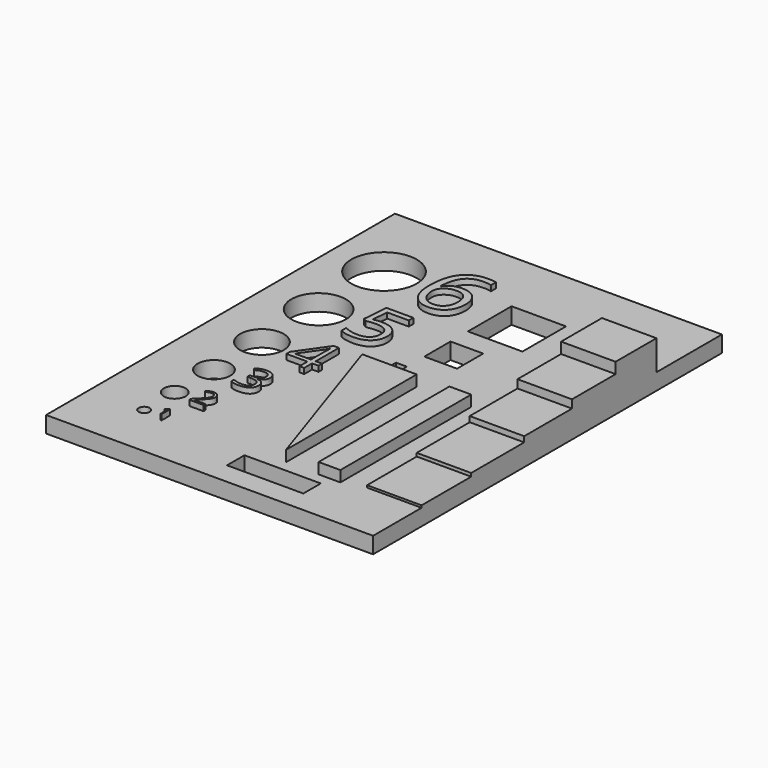
from build123d import *

# Parameters (mm, degrees)
F0_W           = 30
F0_H           = 40
F0_R           = 0.5
F0_R_2         = 1
F0_R_3         = 1.5
F0_R_4         = 2
F0_W_2         = 7
F0_H_2         = 2
F0_R_5         = 2.5
F0_R_6         = 3
F0_W_3         = 1
F0_H_3         = 1
F0_W_4         = 3
F0_H_4         = 3
F0_W_5         = 5
F0_H_5         = 5
F1_DEPTH       = 1.5
F3_DEPTH       = 5
F4_TEXT_SIZE   = 8.3333333333
F4_TEXT_SIZE_2 = 6.9444444444
F4_TEXT_SIZE_3 = 5.5555555556
F4_TEXT_SIZE_4 = 4.1666666667
F4_TEXT_SIZE_5 = 2.7777777778
F4_TEXT_SIZE_6 = 1.3888888889
F5_DEPTH       = 0.5
F6_W           = 2
F6_H           = 15
F7_DEPTH       = 1


# Not quite as in the source:
# - Text() gives the source's letters only with a copy of the font that has no kerning and outlines rounded to 1/6400 em; it was checked with that copy


with BuildPart() as f1:
    # F0 (on Top) → F1 (new body)
    with BuildSketch(Plane.XY):
        Rectangle(F0_W, F0_H)
        with Locations((-10, -15)):
            Circle(F0_R, mode=Mode.SUBTRACT)
        with Locations((-10, -11.5)):
            Circle(F0_R_2, mode=Mode.SUBTRACT)
        with Locations((-10, -7)):
            Circle(F0_R_3, mode=Mode.SUBTRACT)
        with Locations((-10, -1.5)):
            Circle(F0_R_4, mode=Mode.SUBTRACT)
        with Locations((3.5, -17)):
            Rectangle(F0_W_2, F0_H_2, mode=Mode.SUBTRACT)
        with Locations((-10, 5)):
            Circle(F0_R_5, mode=Mode.SUBTRACT)
        with Locations((-10, 12.5)):
            Circle(F0_R_6, mode=Mode.SUBTRACT)
        with Locations((0, 1.5)):
            Rectangle(F0_W_3, F0_H_3, mode=Mode.SUBTRACT)
        with Locations((2, 5.5)):
            Rectangle(F0_W_4, F0_H_4, mode=Mode.SUBTRACT)
        with Locations((3, 11.5)):
            Rectangle(F0_W_5, F0_H_5, mode=Mode.SUBTRACT)
    extrude(amount=F1_DEPTH)

    # F2 (on face) → F3 (join)
    with BuildSketch(Plane.YZ.offset(15)):
        Polygon((-14.4414585084, 1.7), (-14.4414585084, 1.5), (12.4905221164, 1.5), (12.4905221164, 4.25), (7.8079160303, 4.25), (7.8079160303, 3.25), (2.8068085667, 3.25), (2.8068085667, 2.5), (-2.6734757703, 2.5), (-2.6734757703, 2), (-8.7513085455, 2), (-8.7513085455, 1.7), align=None)
    extrude(amount=-F3_DEPTH)

    # F4 (on face) → F5 (join)
    with BuildSketch(Plane.XY.offset(1.5)):
        with Locations((-6, 9.5)):
            Text('6', F4_TEXT_SIZE, font='Open Sans', text_align=(TextAlign.LEFT, TextAlign.BOTTOM))
        with Locations((-6.5, 2.5)):
            Text('5', F4_TEXT_SIZE_2, font='Open Sans', text_align=(TextAlign.LEFT, TextAlign.BOTTOM))
        with Locations((-7, -3.5)):
            Text('4', F4_TEXT_SIZE_3, font='Open Sans', text_align=(TextAlign.LEFT, TextAlign.BOTTOM))
        with Locations((-7.5, -8.5)):
            Text('3', F4_TEXT_SIZE_4, font='Open Sans', text_align=(TextAlign.LEFT, TextAlign.BOTTOM))
        with Locations((-8, -12.5)):
            Text('2', F4_TEXT_SIZE_5, font='Open Sans', text_align=(TextAlign.LEFT, TextAlign.BOTTOM))
        with Locations((-8.5, -15.5)):
            Text('1', F4_TEXT_SIZE_6, font='Open Sans', text_align=(TextAlign.LEFT, TextAlign.BOTTOM))
    extrude(amount=F5_DEPTH)

    # F6 (on face) → F7 (join)
    with BuildSketch(Plane.XY.offset(1.5)):
        Polygon((-2, 0), (3, -15), (3, 0), align=None)
        with Locations((7, -7.5)):
            Rectangle(F6_W, F6_H)
    extrude(amount=F7_DEPTH)


solid = f1.part
